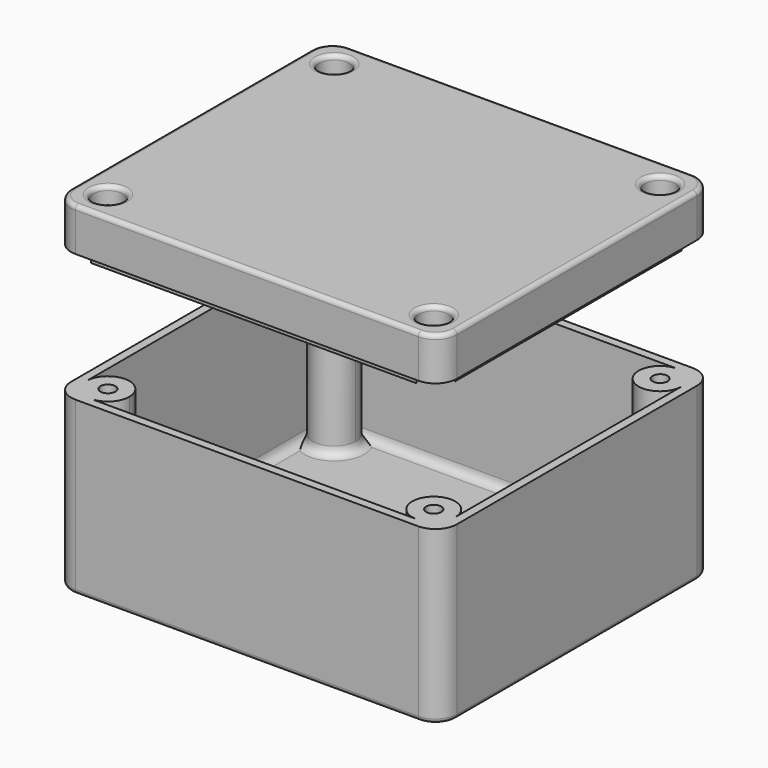
from build123d import *

# Parameters (mm, degrees)
F1_DEPTH      = 2
F0_R          = 1.75
F2_DEPTH      = 40
F3_DEPTH      = 10
F5_R          = 3.5
F6_DEPTH      = 10
F5_R_2        = 2
F7_DEPTH      = 10
F8_DEPTH      = 4
F9_DEPTH      = 12
F10_DEPTH     = 2
F11_T1_DEPTH  = 86
F11_T3_DEPTH  = 76
F11_T6_ANGLE  = 359.64
F11_T8_ANGLE  = 359.64
F11_T10_ANGLE = 359.64
F11_T12_ANGLE = 359.64
F12_R         = 1
F13_R         = 2
F14_R         = 1


# Not quite as in the source:
# - a fillet or chamfer that OpenCascade refuses, or shapes differently, is made with other operations: its cross-section is extruded or revolved along the edge and cut away or added


with BuildPart() as f1:
    # F0 (on Top) → F1 (new body)
    with BuildSketch(Plane.XY):
        with BuildLine():
            Line((-38, -38), (38, -38))
            ThreePointArc((38, -38), (34.4644660941, -29.4644660941), (43, -33))
            Line((43, -33), (43, 33))
            ThreePointArc((43, 33), (34.4644660941, 29.4644660941), (38, 38))
            Line((38, 38), (-38, 38))
            ThreePointArc((-38, 38), (-34.4644660941, 36.5355339059), (-33, 33))
            ThreePointArc((-33, 33), (-38, 28), (-43, 33))
            Line((-43, 33), (-43, -33))
            ThreePointArc((-43, -33), (-38, -28), (-33, -33))
            ThreePointArc((-33, -33), (-34.4644660941, -36.5355339059), (-38, -38))
        make_face()
    extrude(amount=F1_DEPTH)

    # F0 (on Top) → F2 (join)
    with BuildSketch(Plane.XY):
        with BuildLine():
            ThreePointArc((45, 35), (43.5355339059, 38.5355339059), (40, 40))
            Line((40, 40), (-40, 40))
            ThreePointArc((-40, 40), (-43.5355339059, 38.5355339059), (-45, 35))
            Line((-45, 35), (-45, -35))
            ThreePointArc((-45, -35), (-43.5355339059, -38.5355339059), (-40, -40))
            Line((-40, -40), (40, -40))
            ThreePointArc((40, -40), (43.5355339059, -38.5355339059), (45, -35))
            Line((45, -35), (45, 35))
        make_face()
        with BuildLine():
            ThreePointArc((43, -33), (41.5355339059, -36.5355339059), (38, -38))
            Line((38, -38), (-38, -38))
            ThreePointArc((-38, -38), (-41.5355339059, -36.5355339059), (-43, -33))
            Line((-43, -33), (-43, 33))
            ThreePointArc((-43, 33), (-41.5355339059, 36.5355339059), (-38, 38))
            Line((-38, 38), (38, 38))
            ThreePointArc((38, 38), (41.5355339059, 36.5355339059), (43, 33))
            Line((43, 33), (43, -33))
        make_face(mode=Mode.SUBTRACT)
        with BuildLine():
            ThreePointArc((-38, 38), (-41.5355339059, 36.5355339059), (-43, 33))
            ThreePointArc((-43, 33), (-38, 28), (-33, 33))
            ThreePointArc((-33, 33), (-34.4644660941, 36.5355339059), (-38, 38))
        make_face()
        with Locations((-38, 33)):
            Circle(F0_R, mode=Mode.SUBTRACT)
        with BuildLine():
            ThreePointArc((-43, -33), (-41.5355339059, -36.5355339059), (-38, -38))
            ThreePointArc((-38, -38), (-34.4644660941, -36.5355339059), (-33, -33))
            ThreePointArc((-33, -33), (-38, -28), (-43, -33))
        make_face()
        with Locations((-38, -33)):
            Circle(F0_R, mode=Mode.SUBTRACT)
        with BuildLine():
            ThreePointArc((43, -33), (34.4644660941, -29.4644660941), (38, -38))
            ThreePointArc((38, -38), (41.5355339059, -36.5355339059), (43, -33))
        make_face()
        with Locations((38, -33)):
            Circle(F0_R, mode=Mode.SUBTRACT)
        with BuildLine():
            ThreePointArc((38, 38), (34.4644660941, 29.4644660941), (43, 33))
            ThreePointArc((43, 33), (41.5355339059, 36.5355339059), (38, 38))
        make_face()
        with Locations((38, 33)):
            Circle(F0_R, mode=Mode.SUBTRACT)
    extrude(amount=F2_DEPTH)

    # F0 (on Top) → F3 (join)
    with BuildSketch(Plane.XY):
        with Locations((38, 33)):
            Circle(F0_R)
        with Locations((38, -33)):
            Circle(F0_R)
        with Locations((-38, -33)):
            Circle(F0_R)
        with Locations((-38, 33)):
            Circle(F0_R)
    extrude(amount=F3_DEPTH)

    # F11: fillet of radius 2 on 8 edges, made by hand

    # F11_s2 → F11_t1 (join)
    with BuildSketch(Plane.YZ.offset(-43)):
        with BuildLine():
            ThreePointArc((-36, 2), (-37.4142135624, 2.5857864376), (-38, 4))
            Line((-38, 4), (-38, 2))
            Line((-38, 2), (-36, 2))
        make_face()
        with BuildLine():
            ThreePointArc((36, 2), (37.4142135624, 2.5857864376), (38, 4))
            Line((38, 4), (38, 2))
            Line((38, 2), (36, 2))
        make_face()
    extrude(amount=F11_T1_DEPTH)

    # F11_s4 → F11_t3 (join)
    with BuildSketch(Plane.XZ.offset(-38)):
        with BuildLine():
            ThreePointArc((41, 2), (42.4142135624, 2.5857864376), (43, 4))
            Line((43, 4), (43, 2))
            Line((43, 2), (41, 2))
        make_face()
        with BuildLine():
            ThreePointArc((-41, 2), (-42.4142135624, 2.5857864376), (-43, 4))
            Line((-43, 4), (-43, 2))
            Line((-43, 2), (-41, 2))
        make_face()
    extrude(amount=F11_T3_DEPTH)

    # F11_s5 → F11_t6 (revolve)
    with BuildSketch(Plane(origin=(2.6197054312, 2.6032968317, 0), x_dir=(0, 0, 1), z_dir=(0.7093247296, 0.7048818539, 0))):
        with BuildLine():
            ThreePointArc((2, 57.1932265257), (2.5857864376, 55.7790129633), (4, 55.1932265257))
            Line((4, 55.1932265257), (2, 55.1932265257))
            Line((2, 55.1932265257), (2, 57.1932265257))
        make_face()
    revolve(axis=Axis((38, -33, 2), (0, 0, -1)), revolution_arc=F11_T6_ANGLE)

    # F11_s7 → F11_t8 (revolve)
    with BuildSketch(Plane(origin=(2.3809459605, -2.3959530808, 0), x_dir=(0, 0, 1), z_dir=(-0.7048818539, 0.7093247296, 0))):
        with BuildLine():
            ThreePointArc((2, 57.2154409038), (2.5857864376, 55.8012273415), (4, 55.2154409038))
            Line((4, 55.2154409038), (2, 55.2154409038))
            Line((2, 55.2154409038), (2, 57.2154409038))
        make_face()
    revolve(axis=Axis((38, 33, 2), (0, 0, -1)), revolution_arc=F11_T8_ANGLE)

    # F11_s9 → F11_t10 (revolve)
    with BuildSketch(Plane(origin=(-2.3809459605, -2.3959530808, 0), x_dir=(0, 0, 1), z_dir=(0.7048818539, 0.7093247296, 0))):
        with BuildLine():
            ThreePointArc((2, -57.2154409038), (2.5857864376, -55.8012273415), (4, -55.2154409038))
            Line((4, -55.2154409038), (2, -55.2154409038))
            Line((2, -55.2154409038), (2, -57.2154409038))
        make_face()
    revolve(axis=Axis((-38, 33, 2), (0, 0, 1)), revolution_arc=F11_T10_ANGLE)

    # F11_s11 → F11_t12 (revolve)
    with BuildSketch(Plane(origin=(-2.6197054312, 2.6032968317, 0), x_dir=(0, 0, 1), z_dir=(-0.7093247296, 0.7048818539, 0))):
        with BuildLine():
            ThreePointArc((2, -57.1932265257), (2.5857864376, -55.7790129633), (4, -55.1932265257))
            Line((4, -55.1932265257), (2, -55.1932265257))
            Line((2, -55.1932265257), (2, -57.1932265257))
        make_face()
    revolve(axis=Axis((-38, -33, 2), (0, 0, 1)), revolution_arc=F11_T12_ANGLE)

    # F12
    f12_edges = [f1.edges().sort_by_distance(p)[0] for p in [
        (43.535534, 38.535534, 0),
        (0, 40, 0),
        (-43.535534, 38.535534, 0),
        (-45, 0, 0),
        (-43.535534, -38.535534, 0),
        (0, -40, 0),
        (43.535534, -38.535534, 0),
        (45, 0, 0),
    ]]
    fillet(f12_edges, radius=F12_R)


with BuildPart() as f6:
    # F5 (on offset) → F6 (new body)
    with BuildSketch(Plane.XY.offset(79.9)):
        with BuildLine():
            Line((40, 40), (-40, 40))
            ThreePointArc((-40, 40), (-43.5355339059, 38.5355339059), (-45, 35))
            Line((-45, 35), (-45, -35))
            ThreePointArc((-45, -35), (-43.5355339059, -38.5355339059), (-40, -40))
            Line((-40, -40), (40, -40))
            ThreePointArc((40, -40), (43.5355339059, -38.5355339059), (45, -35))
            Line((45, -35), (45, 35))
            ThreePointArc((45, 35), (43.5355339059, 38.5355339059), (40, 40))
        make_face()
        with BuildLine():
            ThreePointArc((-43, 33), (-41.5355339059, 36.5355339059), (-38, 38))
            Line((-38, 38), (38, 38))
            ThreePointArc((38, 38), (41.5355339059, 36.5355339059), (43, 33))
            Line((43, 33), (43, -33))
            ThreePointArc((43, -33), (41.5355339059, -36.5355339059), (38, -38))
            Line((38, -38), (-38, -38))
            ThreePointArc((-38, -38), (-41.5355339059, -36.5355339059), (-43, -33))
            Line((-43, -33), (-43, 33))
        make_face(mode=Mode.SUBTRACT)
        with BuildLine():
            ThreePointArc((-34.2436720058, 36.3), (-35.9384471872, 37.5552167896), (-38, 38))
            ThreePointArc((-38, 38), (-41.5355339059, 36.5355339059), (-43, 33))
            ThreePointArc((-43, 33), (-42.5552167896, 30.9384471872), (-41.3, 29.2436720058))
            ThreePointArc((-41.3, 29.2436720058), (-35.9384471872, 28.4447832104), (-33, 33))
            ThreePointArc((-33, 33), (-33.3212373446, 34.763286708), (-34.2436720058, 36.3))
        make_face()
        with Locations((-38, 33)):
            Circle(F5_R, mode=Mode.SUBTRACT)
        with BuildLine():
            ThreePointArc((-41.3, -29.2436720058), (-42.5552167896, -30.9384471872), (-43, -33))
            ThreePointArc((-43, -33), (-41.5355339059, -36.5355339059), (-38, -38))
            ThreePointArc((-38, -38), (-35.9384471872, -37.5552167896), (-34.2436720058, -36.3))
            ThreePointArc((-34.2436720058, -36.3), (-33.3212373446, -34.763286708), (-33, -33))
            ThreePointArc((-33, -33), (-35.9384471872, -28.4447832104), (-41.3, -29.2436720058))
        make_face()
        with Locations((-38, -33)):
            Circle(F5_R, mode=Mode.SUBTRACT)
        with BuildLine():
            ThreePointArc((38, -38), (41.5355339059, -36.5355339059), (43, -33))
            ThreePointArc((43, -33), (42.5552167896, -30.9384471872), (41.3, -29.2436720058))
            ThreePointArc((41.3, -29.2436720058), (34.4644660941, -29.4644660941), (34.2436720058, -36.3))
            ThreePointArc((34.2436720058, -36.3), (35.9384471872, -37.5552167896), (38, -38))
        make_face()
        with Locations((38, -33)):
            Circle(F5_R, mode=Mode.SUBTRACT)
        with BuildLine():
            ThreePointArc((43, 33), (41.5355339059, 36.5355339059), (38, 38))
            ThreePointArc((38, 38), (35.9384471872, 37.5552167896), (34.2436720058, 36.3))
            ThreePointArc((34.2436720058, 36.3), (34.4644660941, 29.4644660941), (41.3, 29.2436720058))
            ThreePointArc((41.3, 29.2436720058), (42.5552167896, 30.9384471872), (43, 33))
        make_face()
        with Locations((38, 33)):
            Circle(F5_R, mode=Mode.SUBTRACT)
    extrude(amount=-F6_DEPTH)

    # F5 (on offset) → F7 (join)
    with BuildSketch(Plane.XY.offset(79.9)):
        with Locations((-38, 33)):
            Circle(F5_R)
        with Locations((-38, 33)):
            Circle(F5_R_2, mode=Mode.SUBTRACT)
        with Locations((-38, -33)):
            Circle(F5_R)
        with Locations((-38, -33)):
            Circle(F5_R_2, mode=Mode.SUBTRACT)
        with Locations((38, -33)):
            Circle(F5_R)
        with Locations((38, -33)):
            Circle(F5_R_2, mode=Mode.SUBTRACT)
        with Locations((38, 33)):
            Circle(F5_R)
        with Locations((38, 33)):
            Circle(F5_R_2, mode=Mode.SUBTRACT)
    extrude(amount=-F7_DEPTH)

    # F5 (on offset) → F8 (cut)
    with BuildSketch(Plane.XY.offset(79.9)):
        with Locations((-38, 33)):
            Circle(F5_R)
        with Locations((-38, 33)):
            Circle(F5_R_2, mode=Mode.SUBTRACT)
        with Locations((-38, -33)):
            Circle(F5_R)
        with Locations((-38, -33)):
            Circle(F5_R_2, mode=Mode.SUBTRACT)
        with Locations((38, -33)):
            Circle(F5_R)
        with Locations((38, -33)):
            Circle(F5_R_2, mode=Mode.SUBTRACT)
        with Locations((38, 33)):
            Circle(F5_R)
        with Locations((38, 33)):
            Circle(F5_R_2, mode=Mode.SUBTRACT)
    extrude(amount=-F8_DEPTH, mode=Mode.SUBTRACT)

    # F5 (on offset) → F9 (join)
    with BuildSketch(Plane.XY.offset(79.9)):
        with BuildLine():
            Line((38, 38), (-38, 38))
            ThreePointArc((-38, 38), (-35.9384471872, 37.5552167896), (-34.2436720058, 36.3))
            Line((-34.2436720058, 36.3), (34.2436720058, 36.3))
            ThreePointArc((34.2436720058, 36.3), (35.9384471872, 37.5552167896), (38, 38))
        make_face()
        with BuildLine():
            ThreePointArc((-41.3, 29.2436720058), (-42.5552167896, 30.9384471872), (-43, 33))
            Line((-43, 33), (-43, -33))
            ThreePointArc((-43, -33), (-42.5552167896, -30.9384471872), (-41.3, -29.2436720058))
            Line((-41.3, -29.2436720058), (-41.3, 29.2436720058))
        make_face()
        with BuildLine():
            ThreePointArc((-34.2436720058, -36.3), (-35.9384471872, -37.5552167896), (-38, -38))
            Line((-38, -38), (38, -38))
            ThreePointArc((38, -38), (35.9384471872, -37.5552167896), (34.2436720058, -36.3))
            Line((34.2436720058, -36.3), (-34.2436720058, -36.3))
        make_face()
        with BuildLine():
            Line((43, -33), (43, 33))
            ThreePointArc((43, 33), (42.5552167896, 30.9384471872), (41.3, 29.2436720058))
            Line((41.3, 29.2436720058), (41.3, -29.2436720058))
            ThreePointArc((41.3, -29.2436720058), (42.5552167896, -30.9384471872), (43, -33))
        make_face()
    extrude(amount=-F9_DEPTH)

    # F5 (on offset) → F10 (join)
    with BuildSketch(Plane.XY.offset(79.9)):
        with BuildLine():
            Line((34.2436720058, 36.3), (-34.2436720058, 36.3))
            ThreePointArc((-34.2436720058, 36.3), (-33.3212373446, 34.763286708), (-33, 33))
            ThreePointArc((-33, 33), (-35.9384471872, 28.4447832104), (-41.3, 29.2436720058))
            Line((-41.3, 29.2436720058), (-41.3, -29.2436720058))
            ThreePointArc((-41.3, -29.2436720058), (-35.9384471872, -28.4447832104), (-33, -33))
            ThreePointArc((-33, -33), (-33.3212373446, -34.763286708), (-34.2436720058, -36.3))
            Line((-34.2436720058, -36.3), (34.2436720058, -36.3))
            ThreePointArc((34.2436720058, -36.3), (34.4644660941, -29.4644660941), (41.3, -29.2436720058))
            Line((41.3, -29.2436720058), (41.3, 29.2436720058))
            ThreePointArc((41.3, 29.2436720058), (34.4644660941, 29.4644660941), (34.2436720058, 36.3))
        make_face()
    extrude(amount=-F10_DEPTH)

    # F13
    f13_edges = [f6.edges().sort_by_distance(p)[0] for p in [
        (0, 36.3, 77.9),
        (-34.464466, 29.464466, 77.9),
        (-41.3, 0, 77.9),
        (-34.464466, -29.464466, 77.9),
        (0, -36.3, 77.9),
        (34.464466, -29.464466, 77.9),
        (41.3, 0, 77.9),
        (34.464466, 29.464466, 77.9),
    ]]
    fillet(f13_edges, radius=F13_R)

    # F14
    f14_edges = [f6.edges().sort_by_distance(p)[0] for p in [
        (45, 0, 79.9),
        (43.535534, 38.535534, 79.9),
        (0, 40, 79.9),
        (-43.535534, 38.535534, 79.9),
        (-45, 0, 79.9),
        (-43.535534, -38.535534, 79.9),
        (0, -40, 79.9),
        (43.535534, -38.535534, 79.9),
        (-41.5, -33, 79.9),
        (34.5, -33, 79.9),
        (-41.5, 33, 79.9),
        (34.5, 33, 79.9),
    ]]
    fillet(f14_edges, radius=F14_R)


solid = Compound([f1.part, f6.part])
